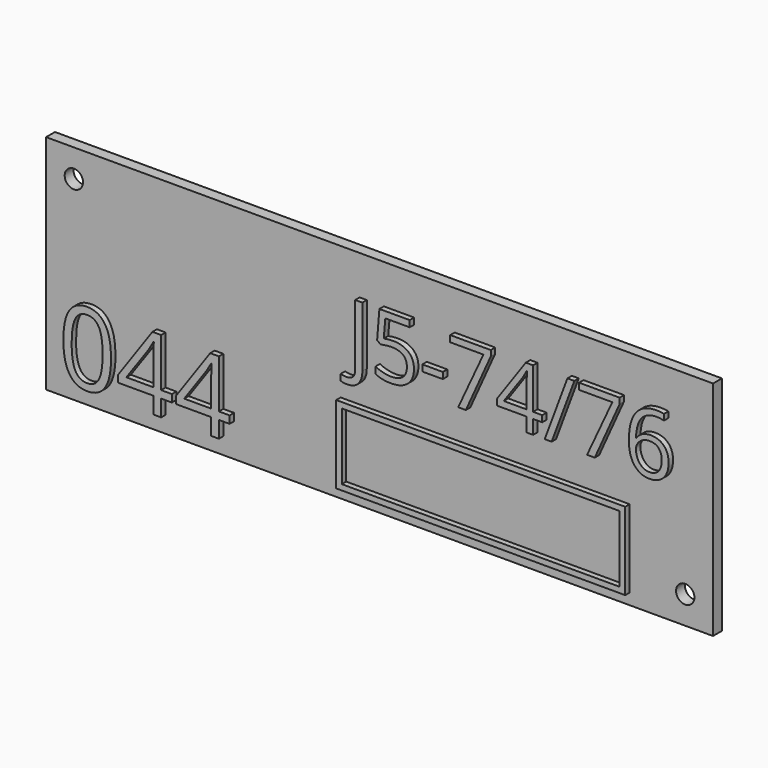
from build123d import *

# Parameters (mm, degrees)
F0_W         = 120
F0_H         = 40
F1_DEPTH     = 2
F3_D         = 3.3
F4_TEXT_SIZE = 15.3501758874
F5_DEPTH     = 1
F6_TEXT_SIZE = 18.1818181818
F7_DEPTH     = 1
F8_W         = 52
F8_H         = 14
F8_W_2       = 49.99999962
F8_H_2       = 11.99999962
F9_DEPTH     = 1


# Not quite as in the source:
# - Text() gives the source's letters only with a copy of the font that has no kerning and outlines rounded to 1/6400 em; it was checked with that copy


with BuildPart() as f1:
    # F0 (on Front) → F1 (new body)
    with BuildSketch(Plane.XZ):
        Rectangle(F0_W, F0_H)
    extrude(amount=F1_DEPTH)

    # F3 (through all)
    with Locations(Plane.XZ.offset(2)):
        with Locations((-55, 15), (55, -15)):
            Hole(F3_D / 2)

    # F4 (on face) → F5 (join)
    with BuildSketch(Plane.XZ.offset(2)):
        with Locations((-5, 2)):
            Text('J5-74/76', F4_TEXT_SIZE, font='Open Sans', text_align=(TextAlign.LEFT, TextAlign.BOTTOM))
    extrude(amount=F5_DEPTH)

    # F6 (on face) → F7 (join)
    with BuildSketch(Plane.XZ.offset(2)):
        with Locations((-57, -17)):
            Text('044', F6_TEXT_SIZE, font='Open Sans', text_align=(TextAlign.LEFT, TextAlign.BOTTOM))
    extrude(amount=F7_DEPTH)

    # F8 (on face) → F9 (join)
    with BuildSketch(Plane.XZ.offset(2)):
        with Locations((19, -11)):
            Rectangle(F8_W, F8_H)
        with Locations((19, -11)):
            Rectangle(F8_W_2, F8_H_2, mode=Mode.SUBTRACT)
    extrude(amount=F9_DEPTH)


solid = f1.part
